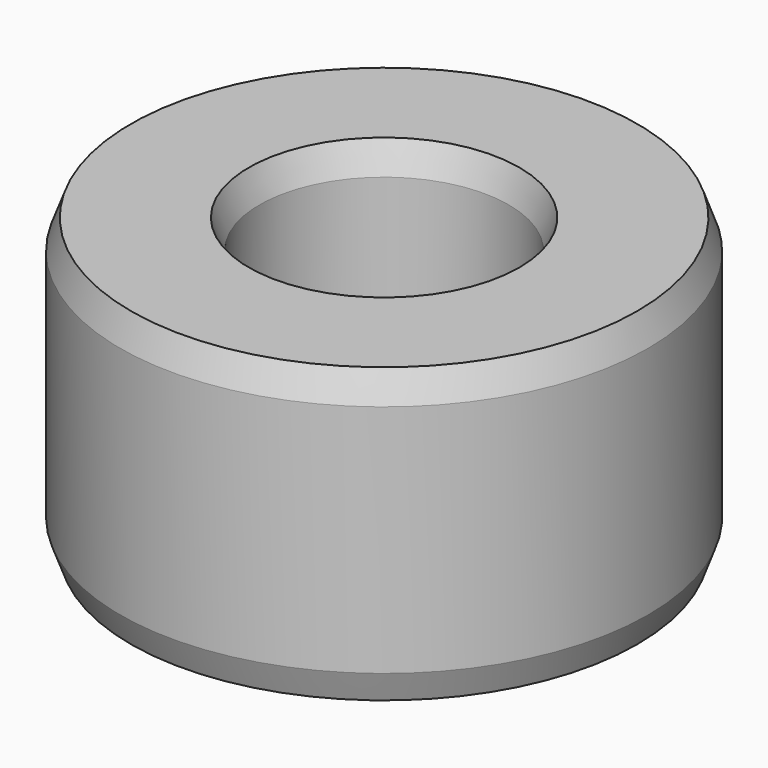
from build123d import *

# Parameters (mm, degrees)
F0_R     = 9
F0_R_2   = 4.25
F1_DEPTH = 10
F2_SIZE2 = 0.3639702343
F2_SIZE  = 1
F3_SIZE2 = 0.3639702343
F3_SIZE  = 1
F4_SIZE2 = 0.3639702343
F4_SIZE  = 1
F5_SIZE2 = 0.3639702343
F5_SIZE  = 1


with BuildPart() as f1:
    # F0 (on Top) → F1 (new body)
    with BuildSketch(Plane.XY):
        Circle(F0_R)
        Circle(F0_R_2, mode=Mode.SUBTRACT)
    extrude(amount=F1_DEPTH)

    # F2
    f2_edges = [f1.edges().sort_by_distance(p)[0] for p in [
        (-4.25, 0, 10),
    ]]
    f2_side = f1.faces().sort_by_distance((-4.25, 0, 5))[0]
    chamfer(f2_edges, length=F2_SIZE, length2=F2_SIZE2, reference=f2_side)

    # F3
    f3_edges = [f1.edges().sort_by_distance(p)[0] for p in [
        (-9, 0, 10),
    ]]
    f3_side = f1.faces().sort_by_distance((-9, 0, 5))[0]
    chamfer(f3_edges, length=F3_SIZE, length2=F3_SIZE2, reference=f3_side)

    # F4
    f4_edges = [f1.edges().sort_by_distance(p)[0] for p in [
        (-9, 0, 0),
    ]]
    f4_side = f1.faces().sort_by_distance((-9, 0, 4.5))[0]
    chamfer(f4_edges, length=F4_SIZE, length2=F4_SIZE2, reference=f4_side)

    # F5
    f5_edges = [f1.edges().sort_by_distance(p)[0] for p in [
        (-4.25, 0, 0),
    ]]
    f5_side = f1.faces().sort_by_distance((-8.391766, 0, 0))[0]
    chamfer(f5_edges, length=F5_SIZE, length2=F5_SIZE2, reference=f5_side)


solid = f1.part
